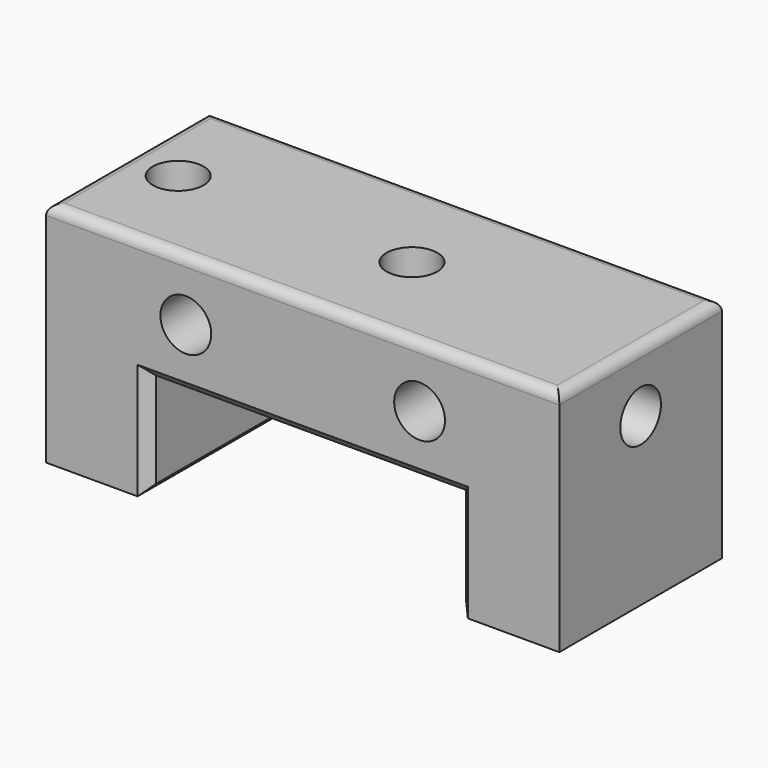
from build123d import *

# Parameters (mm, degrees)
F1_DEPTH = 10
F3_D     = 5
F3_DEPTH = 8
F3_TIP   = 1.5021515476
F5_D     = 4.2
F5_DEPTH = 9.2
F5_TIP   = 1.2618073
F7_D     = 5
F9_D     = 5
F9_DEPTH = 9
F9_TIP   = 1.5021515476
F10_SIZE = 1
F11_R    = 1


# Not quite as in the source:
# - a feature names something its author has since deleted; it is built from what else it names


with BuildPart() as f1:
    # F0 (on Front) → F1 (new body, symmetric)
    with BuildSketch(Plane.XZ):
        Polygon((-25.25, 0), (-25.25, -22.4), (-15.25, -22.4), (-15.25, -12), (15.25, -12), (15.25, -22.4), (25.25, -22.4), (25.25, 0), align=None)
    extrude(amount=F1_DEPTH, both=True)

    # F3
    with Locations(Plane.YZ.offset(25.25)):
        with Locations((0, -6)):
            Hole(F3_D / 2, depth=F3_DEPTH)
            with Locations((0, 0, -(F3_DEPTH + F3_TIP / 2))):  # 118° drill point
                Cone(0, F3_D / 2, F3_TIP, mode=Mode.SUBTRACT)

    # F5
    with Locations(Plane(origin=(0, 0, -22.4), x_dir=(1, 0, 0), z_dir=(0, 0, -1))):
        with Locations((-20.25, 0), (20.25, 0)):
            Hole(F5_D / 2, depth=F5_DEPTH)
            with Locations((0, 0, -(F5_DEPTH + F5_TIP / 2))):  # 118° drill point
                Cone(0, F5_D / 2, F5_TIP, mode=Mode.SUBTRACT)

    # F7 (through all)
    with Locations(Plane.XZ.offset(10)):
        with Locations((11.5, -6), (-11.5, -6)):
            Hole(F7_D / 2)

    # F9
    with Locations(Plane.XY):
        with Locations((-20.25, 0), (2.75, 0)):
            Hole(F9_D / 2, depth=F9_DEPTH)
            with Locations((0, 0, -(F9_DEPTH + F9_TIP / 2))):  # 118° drill point
                Cone(0, F9_D / 2, F9_TIP, mode=Mode.SUBTRACT)

    # F10
    f10_edges = [f1.edges().sort_by_distance(p)[0] for p in [
        (15.25, 0, -22.4),
        (-15.25, 0, -22.4),
        (-15.25, -10, -17.2),
        (0, -10, -12),
        (15.25, -10, -17.2),
        (0, 10, -12),
        (-15.25, 10, -17.2),
        (15.25, 10, -17.2),
    ]]
    chamfer(f10_edges, length=F10_SIZE)

    # F11
    f11_edges = [f1.edges().sort_by_distance(p)[0] for p in [
        (0, 10, 0),
        (0, -10, 0),
        (-25.25, 0, 0),
        (25.25, 0, 0),
    ]]
    fillet(f11_edges, radius=F11_R)


solid = f1.part
